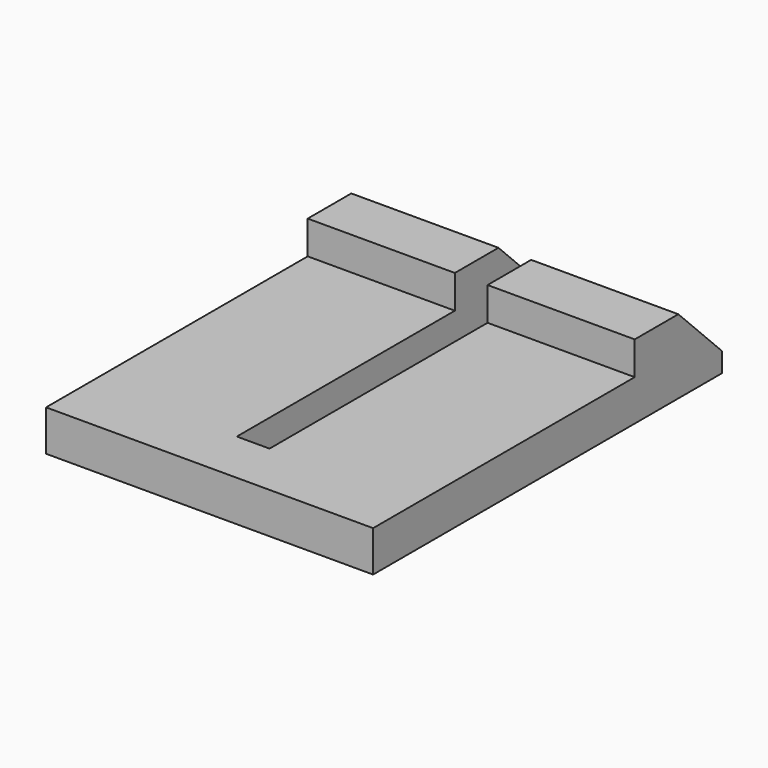
from build123d import *

# Parameters (mm, degrees)
F0_W     = 13.5
F0_H     = 25
F0_W_2   = 1.5
F0_H_2   = 5
F1_DEPTH = 3.75
F0_H_3   = 10
F2_DEPTH = 6.8
F3_SIZE  = 5


with BuildPart() as f1:
    # F0 (on Top) → F1 (new body)
    with BuildSketch(Plane.XY):
        with Locations((-8.25, 17.5)):
            Rectangle(F0_W, F0_H)
        Polygon((1.5, 30), (1.5, 5), (15, 4.9196085972), (15, 30), align=None)
        Polygon((1.5, 5), (1.5, 0), (15, 0), (15, 4.9196085972), align=None)
        with Locations((0.75, 2.5)):
            Rectangle(F0_W_2, F0_H_2)
        with Locations((-0.75, 2.5)):
            Rectangle(F0_W_2, F0_H_2)
        with Locations((-8.25, 2.5)):
            Rectangle(F0_W, F0_H_2)
    extrude(amount=F1_DEPTH)

    # F0 (on Top) → F2 (join)
    with BuildSketch(Plane.XY):
        with Locations((-8.25, 35)):
            Rectangle(F0_W, F0_H_3)
        with Locations((8.25, 35)):
            Rectangle(F0_W, F0_H_3)
    extrude(amount=F2_DEPTH)

    # F3
    f3_edges = [f1.edges().sort_by_distance(p)[0] for p in [
        (-8.25, 40, 6.8),
        (8.25, 40, 6.8),
    ]]
    chamfer(f3_edges, length=F3_SIZE)


solid = f1.part
